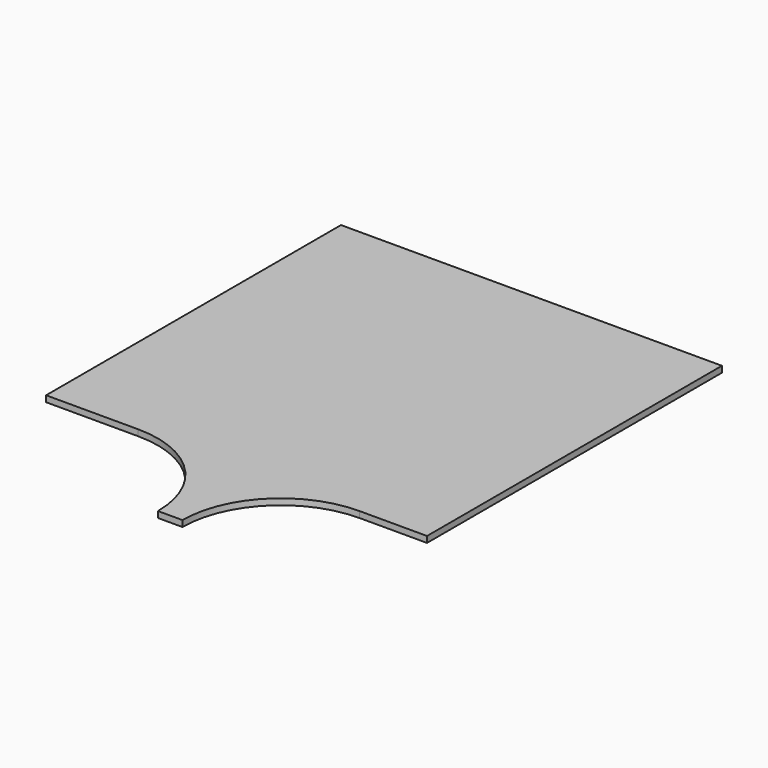
from build123d import *

# Parameters (mm, degrees)
F0_W     = 49.2125
F0_H     = 47.625
F1_DEPTH = 0.79375
F2_W     = 3.175
F2_H     = 12.7
F3_DEPTH = 0.79375
F4_R     = 12.69999


# Not quite as in the source:
# - a fillet or chamfer is up to 0.001 mm smaller than in the source, because OpenCascade refuses the exact size


with BuildPart() as f1:
    # F0 (on Top) → F1 (new body)
    with BuildSketch(Plane.XY):
        with Locations((-36.0471457243, -42.5785098099)):
            Rectangle(F0_W, F0_H)
    extrude(amount=F1_DEPTH)

    # F2 (on face) → F3 (join)
    with BuildSketch(Plane.XY.offset(0.79375)):
        with Locations((-34.4596457243, -72.7410098099)):
            Rectangle(F2_W, F2_H)
    extrude(amount=-F3_DEPTH)

    # F4 (radius 12.7 in the source; OpenCascade refuses exactly that, so slightly less here)
    f4_edges = [f1.edges().sort_by_distance(p)[0] for p in [
        (-36.047146, -66.39101, 0.396875),
        (-32.872146, -66.39101, 0.396875),
    ]]
    fillet(f4_edges, radius=F4_R)


solid = f1.part
